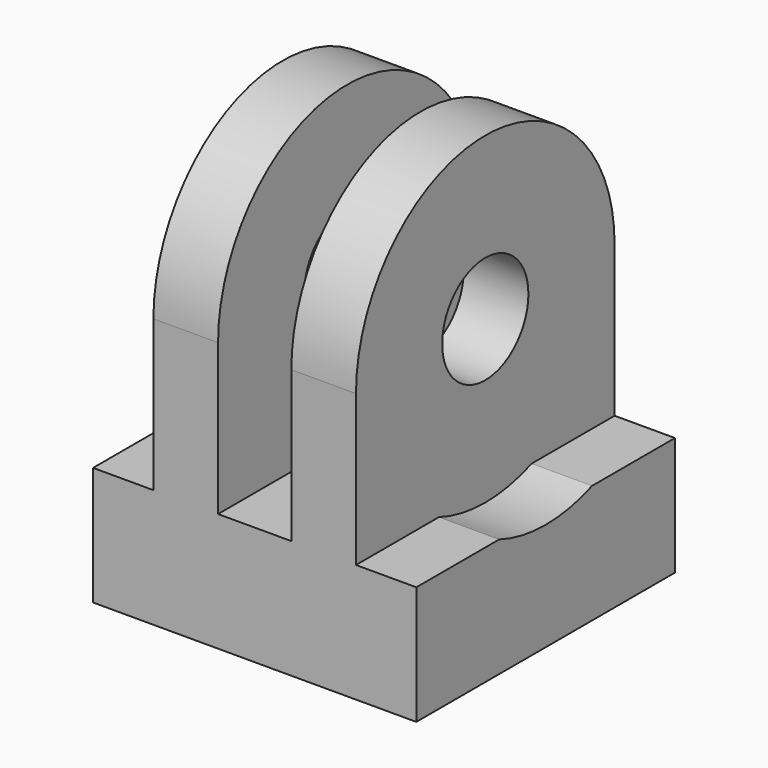
from build123d import *

# Parameters (mm, degrees)
F0_R     = 2.5
F1_DEPTH = 7.5
F2_W     = 3.4
F2_H     = 15.4505071864
F2_W_2   = 3.8797123611
F2_W_3   = 3.8316924378
F3_DEPTH = 16.41578
F5_DEPTH = 2.8
F7_DEPTH = 2.8


with BuildPart() as f1:
    # F0 (on Right) → F1 (new body, symmetric)
    with BuildSketch(Plane.YZ):
        with BuildLine():
            Line((7.5, -12.5), (7.5, 0))
            ThreePointArc((7.5, 0), (0, 7.5), (-7.5, 0))
            Line((-7.5, 0), (-7.5, -12.5))
            Line((-7.5, -12.5), (7.5, -12.5))
        make_face()
        Circle(F0_R, mode=Mode.SUBTRACT)
    extrude(amount=F1_DEPTH, both=True)

    # F2 (on Front) → F3 (cut, symmetric)
    with BuildSketch(Plane.XZ):
        with Locations((0, 0.7252535932)):
            Rectangle(F2_W, F2_H)
        with Locations((-6.6398561805, 0.7252535932)):
            Rectangle(F2_W_2, F2_H)
        with Locations((6.6158462189, 0.7252535932)):
            Rectangle(F2_W_3, F2_H)
    extrude(amount=F3_DEPTH, both=True, mode=Mode.SUBTRACT)

    # F4 (on face) → F5 (cut, through all)
    with BuildSketch(Plane(origin=(-7.5, 0, 0), x_dir=(0, -1, 0), z_dir=(-1, 0, 0))):
        with BuildLine():
            ThreePointArc((2.6925824036, -7), (6.1824092402, -4.2459175671), (7.5, 0))
            ThreePointArc((7.5, 0), (-4.2459175671, 6.1824092402), (-2.6925824036, -7))
            Line((-2.6925824036, -7), (2.6925824036, -7))
        make_face()
        with BuildLine():
            Line((2.6925824036, -7), (-2.6925824036, -7))
            ThreePointArc((-2.6925824036, -7), (0, -7.5), (2.6925824036, -7))
        make_face()
    extrude(amount=-F5_DEPTH, mode=Mode.SUBTRACT)

    # F6 (on face) → F7 (cut, through all)
    with BuildSketch(Plane.YZ.offset(7.5)):
        with BuildLine():
            Line((2.6925824036, -7), (-2.6925824036, -7))
            ThreePointArc((-2.6925824036, -7), (0, -7.5), (2.6925824036, -7))
        make_face()
        with BuildLine():
            ThreePointArc((2.6925824036, -7), (6.1824092402, -4.2459175671), (7.5, 0))
            ThreePointArc((7.5, 0), (-4.2459175671, 6.1824092402), (-2.6925824036, -7))
            Line((-2.6925824036, -7), (2.6925824036, -7))
        make_face()
    extrude(amount=-F7_DEPTH, mode=Mode.SUBTRACT)


solid = f1.part
